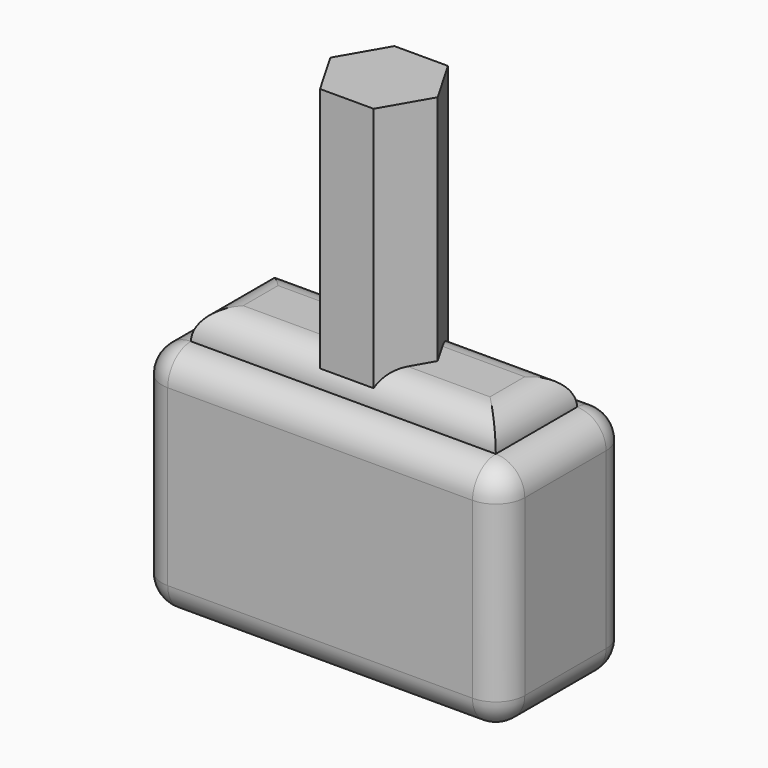
from build123d import *

# Parameters (mm, degrees)
F1_DEPTH      = 17
F3_START      = -1
F2_W          = 25
F2_H          = 11
F2_W_2        = 21
F2_H_2        = 7
F3_DEPTH      = 16
F4_DEPTH      = 1
F4_DEPTH_BACK = 2
F5_R          = 2
F6_R          = 1.99999


# Not quite as in the source:
# - a fillet or chamfer is up to 0.001 mm smaller than in the source, because OpenCascade refuses the exact size


with BuildPart() as f1:
    # F0 (on Top) → F1 (new body)
    with BuildSketch(Plane.XY):
        Polygon((1.8475208614, -3.2), (3.6950417228, 0), (1.8475208614, 3.2), (-1.8475208614, 3.2), (-3.6950417228, 0), (-1.8475208614, -3.2), align=None)
    extrude(amount=F1_DEPTH)


with BuildPart() as f3:
    # F2 (on Top) → F3 (new body)
    with BuildSketch(Plane.XY.offset(F3_START)):
        Rectangle(F2_W, F2_H)
        Rectangle(F2_W_2, F2_H_2, mode=Mode.SUBTRACT)
    extrude(amount=-F3_DEPTH)

    # F6 (radius 2 in the source; OpenCascade refuses exactly that, so slightly less here)
    f6_edges = [f3.edges().sort_by_distance(p)[0] for p in [
        (12.5, 5.5, -9),
        (-12.5, 5.5, -9),
        (0, 5.5, -1),
        (0, 5.5, -17),
        (-12.5, -5.5, -9),
        (12.5, -5.5, -9),
        (0, -5.5, -1),
        (0, -5.5, -17),
        (-12.5, 0, -1),
        (-12.5, 0, -17),
        (12.5, 0, -1),
        (12.5, 0, -17),
    ]]
    fillet(f6_edges, radius=F6_R)


with BuildPart() as f4:
    # F2 (on Top) → F4 (new body, two sides)
    with BuildSketch(Plane.XY) as f4_sk:
        Rectangle(F2_W_2, F2_H_2)
    extrude(amount=F4_DEPTH)
    extrude(f4_sk.sketch, amount=-F4_DEPTH_BACK)

    # F5
    f5_edges = [f4.edges().sort_by_distance(p)[0] for p in [
        (0, -3.5, 1),
        (10.5, 0, 1),
        (0, 3.5, 1),
        (-10.5, 0, 1),
    ]]
    fillet(f5_edges, radius=F5_R)


solid = Compound([f1.part, f3.part, f4.part])
